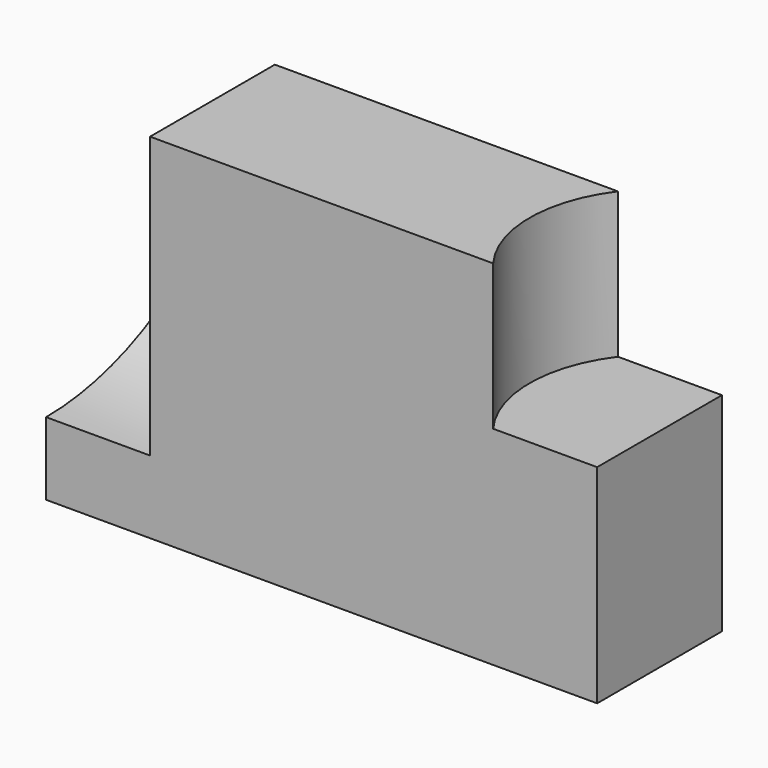
from build123d import *

# Parameters (mm, degrees)
F0_W     = 53
F0_H     = 34
F1_DEPTH = 15
F2_R     = 27
F3_DEPTH = 10
F5_DEPTH = 14


with BuildPart() as f1:
    # F0 (on Front) → F1 (new body)
    with BuildSketch(Plane.XZ):
        with Locations((2.3567589563, 1.288594678)):
            Rectangle(F0_W, F0_H)
    extrude(amount=F1_DEPTH)

    # F2 (on face) → F3 (cut)
    with BuildSketch(Plane(origin=(-24.1432410437, 0, 0), x_dir=(0, -1, 0), z_dir=(-1, 0, 0))):
        with Locations((15, 18.288594678)):
            Circle(F2_R)
    extrude(amount=-F3_DEPTH, mode=Mode.SUBTRACT)

    # F4 (on face) → F5 (cut)
    with BuildSketch(Plane.XY.offset(18.288594678)):
        with BuildLine():
            Line((28.8567589563, 0), (18.8567589563, 0))
            ThreePointArc((18.8567589563, 0), (16.3567589563, -7.5), (18.8567589563, -15))
            Line((18.8567589563, -15), (28.8567589563, -15))
            Line((28.8567589563, -15), (28.8567589563, 0))
        make_face()
    extrude(amount=-F5_DEPTH, mode=Mode.SUBTRACT)


solid = f1.part
